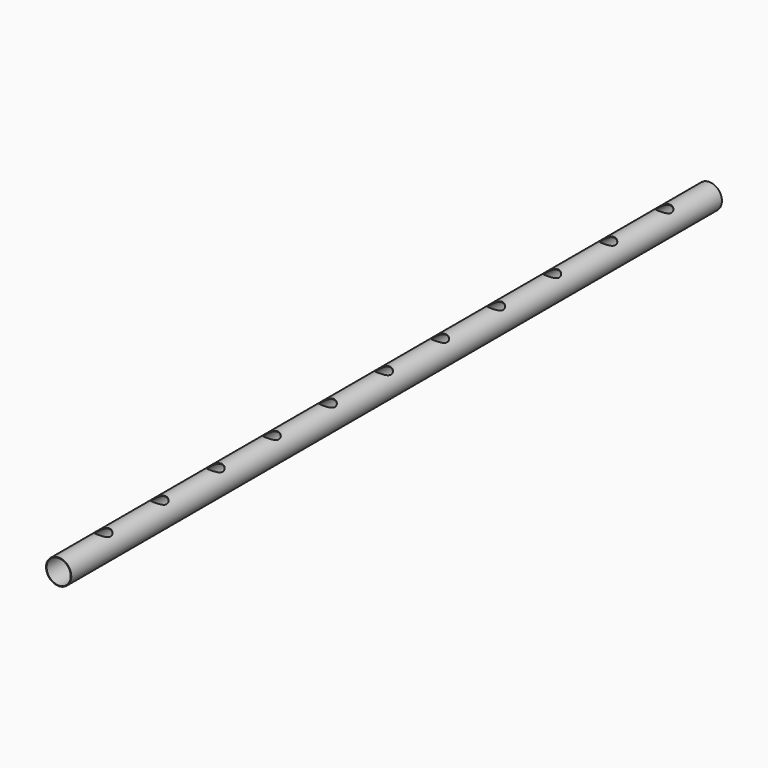
from build123d import *

# Parameters (mm, degrees)
F0_R     = 45
F0_R_2   = 43
F1_DEPTH = 1450
F4_D     = 50
F4_DEPTH = 50
F4_TIP   = 15.0215154757
F6_D     = 0.5
F6_DEPTH = 50
F6_TIP   = 0.1502151548


# Not quite as in the source:
# - a feature names something its author has since deleted; it is built from what else it names


with BuildPart() as f1:
    # F0 (on Front) → F1 (new body, symmetric)
    with BuildSketch(Plane.XZ):
        Circle(F0_R)
        Circle(F0_R_2, mode=Mode.SUBTRACT)
    extrude(amount=F1_DEPTH, both=True)

    # F4
    with Locations(Plane.XY.offset(45)):
        with Locations((0, -1250), (0, -1000), (0, -750), (0, -500), (0, -250), (0, 0), (0, 250), (0, 500), (0, 750), (0, 1000), (0, 1250)):
            Hole(F4_D / 2, depth=F4_DEPTH)
            with Locations((0, 0, -(F4_DEPTH + F4_TIP / 2))):  # 118° drill point
                Cone(0, F4_D / 2, F4_TIP, mode=Mode.SUBTRACT)

    # F6
    with Locations(Plane.XY):
        with Locations((0, 0)):
            Hole(F6_D / 2, depth=F6_DEPTH)
            with Locations((0, 0, -(F6_DEPTH + F6_TIP / 2))):  # 118° drill point
                Cone(0, F6_D / 2, F6_TIP, mode=Mode.SUBTRACT)


solid = f1.part
